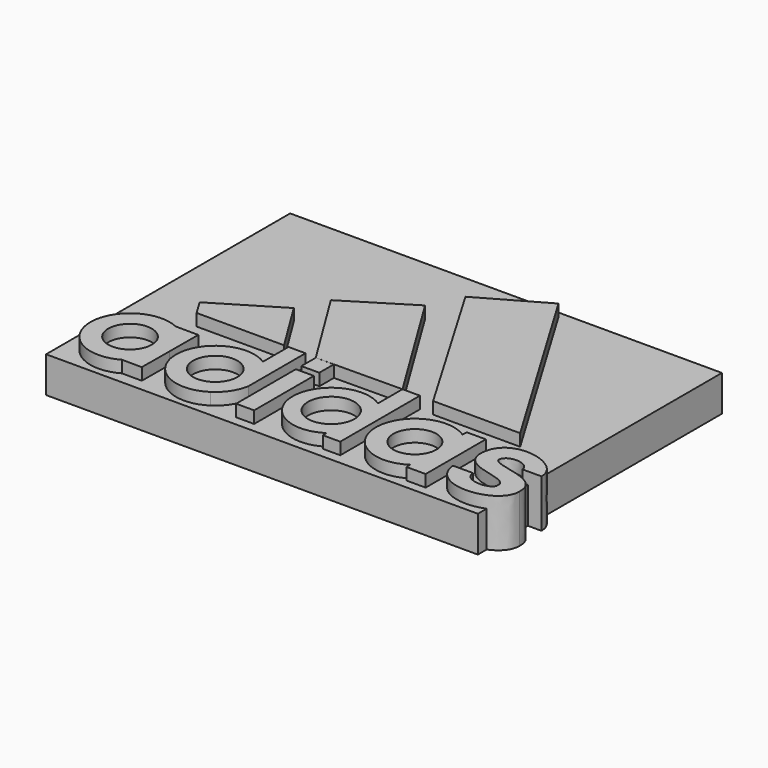
from build123d import *

# Parameters (mm, degrees)
F2_DEPTH = 25.4
F0_R     = 11.5336925559
F0_W     = 9.541330096
F0_H     = 39.5781323314
F0_R_2   = 11.380629632
F0_H_2   = 9.5591302517
F1_W     = 228.8039848208
F1_H     = 161.6584509611
F3_DEPTH = 19.05


with BuildPart() as f2:
    # F0 (on Top) → F2 (new body)
    with BuildSketch(Plane.XY):
        Polygon((-51.0945059359, 34.3518182635), (-84.4939826515, 13.6732111501), (-57.1369986801, -30.5129830238), (-11.4884115756, -30.1327314228), align=None)
    extrude(amount=F2_DEPTH)


with BuildPart() as f2b:
    # F0 (on Top) → F2, piece 2 (new body)
    with BuildSketch(Plane.XY):
        with BuildLine():
            ThreePointArc((-107.9762237087, -63.8860243261), (-107.9759929518, -63.8292248991), (-107.9759160326, -63.7724250555))
            ThreePointArc((-107.9759160326, -63.7724250555), (-111.2166703627, -52.5731037336), (-119.9373394473, -44.8350666817))
            ThreePointArc((-119.9373394473, -44.8350666817), (-149.9052734682, -64.5315465682), (-118.5908724142, -82.0082932916))
            ThreePointArc((-118.5908724142, -82.0082932916), (-110.851541588, -74.3716434809), (-107.9762237087, -63.8860243261))
        make_face()
        with Locations((-128.9474666119, -63.7724250555)):
            Circle(F0_R, mode=Mode.SUBTRACT)
        with BuildLine():
            ThreePointArc((-119.9373394473, -44.8350666817), (-111.2166703627, -52.5731037336), (-107.9759160326, -63.7724250555))
            ThreePointArc((-107.9759160326, -63.7724250555), (-107.9759929518, -63.8292248991), (-107.9762237087, -63.8860243261))
            Line((-107.9762237087, -63.8860243261), (-107.8733798367, -44.9004164099))
            Line((-107.8733798367, -44.9004164099), (-119.9373394473, -44.8350666817))
        make_face()
        with BuildLine():
            Line((-108.074699505, -82.0652587543), (-107.9762237087, -63.8860243261))
            ThreePointArc((-107.9762237087, -63.8860243261), (-110.851541588, -74.3716434809), (-118.5908724142, -82.0082932916))
            Line((-118.5908724142, -82.0082932916), (-108.074699505, -82.0652587543))
        make_face()
    extrude(amount=F2_DEPTH)



with BuildPart() as f2c:
    # F0 (on Top) → F2, piece 3 (new body)
    with BuildSketch(Plane.XY):
        Polygon((-92.0550826628, -1.4315552488), (-125.7108291716, -21.712434453), (-120.7355512429, -29.968816787), (-74.3747093637, -29.968816787), align=None)
    extrude(amount=F2_DEPTH)


with BuildPart() as f2d:
    # F0 (on Top) → F2, piece 4 (new body)
    with BuildSketch(Plane.XY):
        with BuildLine():
            ThreePointArc((-62.9558414221, -60.6451802377), (-66.0588539194, -52.8699310888), (-71.9823092222, -46.9542009427))
            Line((-71.9823092222, -46.9542009427), (-71.9823092222, -61.4527142385))
            ThreePointArc((-71.9823092222, -61.4527142385), (-71.7219259683, -62.8601804955), (-71.6346996434, -64.2888695002))
            ThreePointArc((-71.6346996434, -64.2888695002), (-71.7219259683, -65.7175585048), (-71.9823092222, -67.1250247618))
            Line((-71.9823092222, -67.1250247618), (-71.9823092222, -81.6235380576))
            ThreePointArc((-71.9823092222, -81.6235380576), (-66.0588539194, -75.7078079115), (-62.9558414221, -67.9325587626))
            Line((-62.9558414221, -67.9325587626), (-62.9558414221, -60.6451802377))
        make_face()
        with BuildLine():
            Line((-62.9558414221, -30.0241652876), (-71.9823092222, -30.0241652876))
            Line((-71.9823092222, -30.0241652876), (-71.9823092222, -46.9542009427))
            ThreePointArc((-71.9823092222, -46.9542009427), (-66.0588539194, -52.8699310888), (-62.9558414221, -60.6451802377))
            Line((-62.9558414221, -60.6451802377), (-62.9558414221, -30.0241652876))
        make_face()
        with BuildLine():
            Line((-71.9823092222, -61.4527142385), (-71.9823092222, -46.9542009427))
            ThreePointArc((-71.9823092222, -46.9542009427), (-104.1239235622, -64.2888695002), (-71.9823092222, -81.6235380576))
            Line((-71.9823092222, -81.6235380576), (-71.9823092222, -67.1250247618))
            ThreePointArc((-71.9823092222, -67.1250247618), (-95.1225710504, -64.2888695002), (-71.9823092222, -61.4527142385))
        make_face()
    extrude(amount=F2_DEPTH)


with BuildPart() as f2e:
    # F0 (on Top) → F2, piece 5 (new body)
    with BuildSketch(Plane.XY):
        with Locations((-52.3663336321, -63.4756200016)):
            Rectangle(F0_W, F0_H)
    extrude(amount=F2_DEPTH)


with BuildPart() as f2f:
    # F0 (on Top) → F2, piece 6 (new body)
    with BuildSketch(Plane.XY):
        with BuildLine():
            Line((-2.2344286554, -30.1327314228), (-11.4884115756, -30.1327314228))
            Line((-11.4884115756, -30.1327314228), (-11.4884115756, -46.3416812132))
            ThreePointArc((-11.4884115756, -46.3416812132), (-4.7290138195, -53.6991112265), (-2.2795860101, -63.3852630854))
            ThreePointArc((-2.2795860101, -63.3852630854), (-4.7290138195, -73.0714149442), (-11.4884115756, -80.4288449576))
            Line((-11.4884115756, -80.4288449576), (-11.4884115756, -82.9032436013))
            Line((-11.4884115756, -82.9032436013), (-2.2344286554, -82.9032436013))
            Line((-2.2344286554, -82.9032436013), (-2.2344286554, -30.1327314228))
        make_face()
        with BuildLine():
            Line((-11.4884115756, -58.2216957499), (-11.4884115756, -46.3416812132))
            ThreePointArc((-11.4884115756, -46.3416812132), (-43.0324647199, -63.3852630854), (-11.4884115756, -80.4288449576))
            Line((-11.4884115756, -80.4288449576), (-11.4884115756, -68.5488304208))
            ThreePointArc((-11.4884115756, -68.5488304208), (-34.959603112, -63.3852630854), (-11.4884115756, -58.2216957499))
        make_face()
        with BuildLine():
            ThreePointArc((-2.2795860101, -63.3852630854), (-4.7290138195, -53.6991112265), (-11.4884115756, -46.3416812132))
            Line((-11.4884115756, -46.3416812132), (-11.4884115756, -58.2216957499))
            ThreePointArc((-11.4884115756, -58.2216957499), (-10.639794053, -60.7417407315), (-10.3524476179, -63.3852630854))
            ThreePointArc((-10.3524476179, -63.3852630854), (-10.639794053, -66.0287854392), (-11.4884115756, -68.5488304208))
            Line((-11.4884115756, -68.5488304208), (-11.4884115756, -80.4288449576))
            ThreePointArc((-11.4884115756, -80.4288449576), (-4.7290138195, -73.0714149442), (-2.2795860101, -63.3852630854))
        make_face()
    extrude(amount=F2_DEPTH)


with BuildPart() as f2g:
    # F0 (on Top) → F2, piece 7 (new body)
    with BuildSketch(Plane.XY):
        with BuildLine():
            Line((33.3248190582, -80.9727901538), (33.3248190582, -46.3803267161))
            ThreePointArc((33.3248190582, -46.3803267161), (1.2023110457, -63.676558435), (33.3248190582, -80.9727901538))
        make_face()
        with Locations((21.920107305, -63.676558435)):
            Circle(F0_R_2, mode=Mode.SUBTRACT)
        with BuildLine():
            ThreePointArc((33.3248190582, -80.9727901538), (40.1616474859, -73.4986403768), (42.6379035644, -63.676558435))
            ThreePointArc((42.6379035644, -63.676558435), (40.1616474859, -53.8544764931), (33.3248190582, -46.3803267161))
            Line((33.3248190582, -46.3803267161), (33.3248190582, -80.9727901538))
        make_face()
        with BuildLine():
            ThreePointArc((33.3248190582, -46.3803267161), (40.1616474859, -53.8544764931), (42.6379035644, -63.676558435))
            ThreePointArc((42.6379035644, -63.676558435), (40.1616474859, -73.4986403768), (33.3248190582, -80.9727901538))
            Line((33.3248190582, -80.9727901538), (33.3248190582, -83.4800675511))
            Line((33.3248190582, -83.4800675511), (43.4636287391, -83.4800675511))
            Line((43.4636287391, -83.4800675511), (43.4636287391, -43.6490178108))
            Line((43.4636287391, -43.6490178108), (33.3248190582, -43.6490178108))
            Line((33.3248190582, -43.6490178108), (33.3248190582, -46.3803267161))
        make_face()
    extrude(amount=F2_DEPTH)


with BuildPart() as f2h:
    # F0 (on Top) → F2, piece 8 (new body)
    with BuildSketch(Plane.XY):
        with BuildLine():
            Line((58.1554566098, -70.5598088785), (47.5999824703, -70.5598088785))
            add(Edge.make_bspline(
                [(47.5999824703, -70.5598088785), (49.5010092854, -90.3848129197), (83.9333076226, -87.0293162841), (83.5507873642, -71.3937439102)],
                knots=[0, 0, 0, 0, 35.9604758055, 35.9604758055, 35.9604758055, 35.9604758055], degree=3))
            add(Edge.make_bspline(
                [(83.5507873642, -71.3937439102), (84.1839209979, -56.8009070249), (60.4972094297, -60.2178759873), (58.9604414999, -54.456923157)],
                knots=[0, 0, 0, 0, 29.8586839454, 29.8586839454, 29.8586839454, 29.8586839454], degree=3))
            add(Edge.make_bspline(
                [(58.9604414999, -54.456923157), (59.7041723272, -48.5431283295), (71.4366002474, -49.1966214378), (72.1989516421, -55.1880527146)],
                knots=[0, 0, 0, 0, 13.2095221181, 13.2095221181, 13.2095221181, 13.2095221181], degree=3))
            Line((72.1989516421, -55.1880527146), (82.1682080838, -55.1880527146))
            add(Edge.make_bspline(
                [(82.1682080838, -55.1880527146), (82.6870746879, -41.6859303163), (52.6399704235, -34.4332249736), (49.8361763634, -52.5753086121)],
                knots=[0, 0, 0, 0, 31.868338701, 31.868338701, 31.868338701, 31.868338701], degree=3))
            add(Edge.make_bspline(
                [(49.8361763634, -52.5753086121), (49.7805065758, -52.9355226367), (49.7355768501, -53.3057479852), (49.7018396854, -53.6861345172)],
                knots=[31.868338701, 31.868338701, 31.868338701, 31.868338701, 32.5010897548, 32.5010897548, 32.5010897548, 32.5010897548], degree=3))
            add(Edge.make_bspline(
                [(49.7018396854, -53.6861345172), (48.3377947774, -69.6180662759), (74.1305380627, -64.2111304974), (73.0244419212, -72.7832366078)],
                knots=[0.6783402198, 0.6783402198, 0.6783402198, 0.6783402198, 30.7580235623, 30.7580235623, 30.7580235623, 30.7580235623], degree=3))
            add(Edge.make_bspline(
                [(58.1554566098, -70.5598088785), (58.8323771954, -78.6550715566), (73.4929313503, -77.367492494), (73.0244419212, -72.7832366078)],
                knots=[0, 0, 0, 0, 15.0343059386, 15.0343059386, 15.0343059386, 15.0343059386], degree=3))
        make_face()
    extrude(amount=F2_DEPTH)


with BuildPart() as f2i:
    # F0 (on Top) → F2, piece 9 (new body)
    with BuildSketch(Plane.XY):
        Polygon((-9.054414928, 70.1610743999), (-42.9158993065, 50.8752018213), (5.0083836541, -30.4661039263), (51.1389710009, -30.4661039263), align=None)
    extrude(amount=F2_DEPTH)


with BuildPart() as f2j:
    # F0 (on Top) → F2, piece 10 (new body)
    with BuildSketch(Plane.XY):
        with Locations((-52.3663336321, -35.2925481497)):
            Rectangle(F0_W, F0_H_2)
    extrude(amount=F2_DEPTH)


with BuildPart() as f2b_1:
    add(f2b.part)

    add(f2c.part)  # F3 merges F2c

    add(f2d.part)  # F3 merges F2d

    add(f2e.part)  # F3 merges F2e

    add(f2f.part)  # F3 merges F2f

    add(f2g.part)  # F3 merges F2g

    add(f2h.part)  # F3 merges F2h

    add(f2i.part)  # F3 merges F2i

    add(f2j.part)  # F3 merges F2j
    # F1 (on Top) → F3 (join)
    with BuildSketch(Plane.XY):
        with Locations((-39.4312478602, -7.4402168393)):
            Rectangle(F1_W, F1_H)
    extrude(amount=F3_DEPTH)


solid = Compound([f2.part, f2b_1.part])
